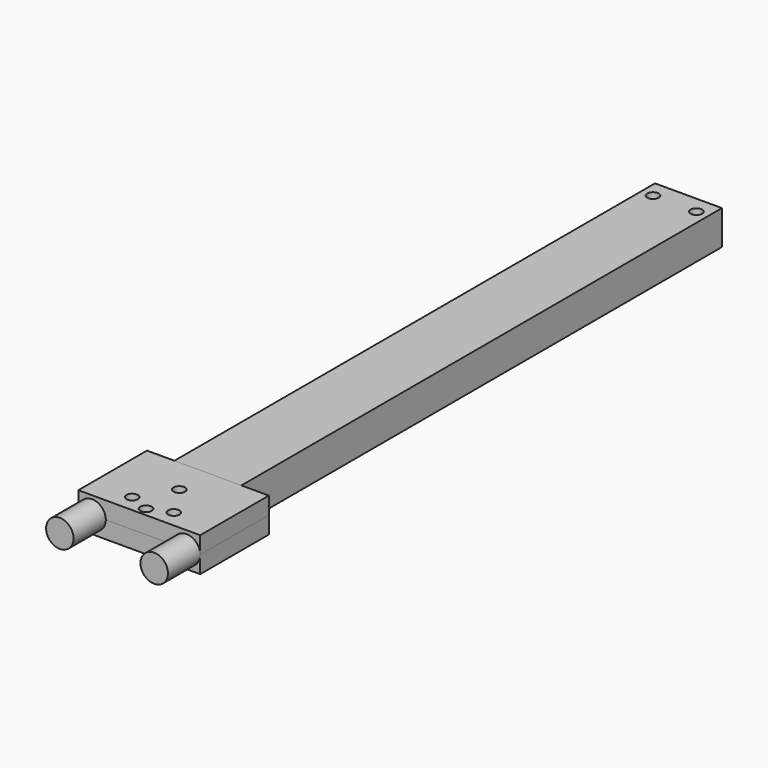
from build123d import *

# Parameters (mm, degrees)
F1_DEPTH   = 11.75
F2_DEPTH   = 25
F3_DEPTH   = 25
F4_DEPTH   = 25
F5_W       = 19.5
F5_H       = 5
F6_DEPTH   = 175
F8_D       = 3.35
F8_DEPTH   = 10
F8_TIP     = 1.0064415369
F8_2_D     = 3.35
F8_2_DEPTH = 10
F8_2_TIP   = 1.0064415369
F8_3_D     = 3.35
F8_3_DEPTH = 10
F8_3_TIP   = 1.0064415369


with BuildPart() as f1:
    # F0 (on Front) → F1 (new body)
    with BuildSketch(Plane.XZ):
        with BuildLine():
            ThreePointArc((-83.867456615, 12.549745962), (-79.867456615, 8.549745962), (-75.867456615, 12.549745962))
            Line((-75.867456615, 12.549745962), (-79.867456615, 12.549745962))
            Line((-79.867456615, 12.549745962), (-83.867456615, 12.549745962))
        make_face()
        with BuildLine():
            Line((-79.867456615, 12.549745962), (-75.867456615, 12.549745962))
            ThreePointArc((-75.867456615, 12.549745962), (-79.867456615, 16.549745962), (-83.867456615, 12.549745962))
            Line((-83.867456615, 12.549745962), (-79.867456615, 12.549745962))
        make_face()
    extrude(amount=F1_DEPTH)


with BuildPart() as f1b:
    # F0 (on Front) → F1, piece 2 (new body)
    with BuildSketch(Plane.XZ):
        with BuildLine():
            ThreePointArc((-103.367456615, 12.549745962), (-107.367456615, 16.549745962), (-111.367456615, 12.549745962))
            Line((-111.367456615, 12.549745962), (-107.367456615, 12.549745962))
            Line((-107.367456615, 12.549745962), (-103.367456615, 12.549745962))
        make_face()
        with BuildLine():
            Line((-107.367456615, 12.549745962), (-111.367456615, 12.549745962))
            ThreePointArc((-111.367456615, 12.549745962), (-107.367456615, 8.549745962), (-103.367456615, 12.549745962))
            Line((-103.367456615, 12.549745962), (-107.367456615, 12.549745962))
        make_face()
    extrude(amount=F1_DEPTH)


with BuildPart() as f2:
    # F0 (on Front) → F2 (new body)
    with BuildSketch(Plane.XZ):
        with BuildLine():
            Line((-75.867456615, 7.549745962), (-75.867456615, 12.549745962))
            ThreePointArc((-75.867456615, 12.549745962), (-79.867456615, 8.549745962), (-83.867456615, 12.549745962))
            Line((-83.867456615, 12.549745962), (-103.367456615, 12.549745962))
            ThreePointArc((-103.367456615, 12.549745962), (-107.367456615, 8.549745962), (-111.367456615, 12.549745962))
            Line((-111.367456615, 12.549745962), (-111.367456615, 7.549745962))
            Line((-111.367456615, 7.549745962), (-75.867456615, 7.549745962))
        make_face()
    extrude(amount=-F2_DEPTH)

    # F8
    with Locations(Plane(origin=(0, 0, 7.549745962), x_dir=(1, 0, 0), z_dir=(0, 0, -1))):
        with Locations((-99.692456615, -5), (-87.542456615, -5), (-99.942456615, -195), (-87.292456615, -195), (-93.617456615, -14.6046723992), (-93.617456615, -2.4546723992)):
            Hole(F8_D / 2, depth=F8_DEPTH)
            with Locations((0, 0, -(F8_DEPTH + F8_TIP / 2))):  # 118° drill point
                Cone(0, F8_D / 2, F8_TIP, mode=Mode.SUBTRACT)


with BuildPart() as f3:
    # F0 (on Front) → F3 (new body)
    with BuildSketch(Plane.XZ):
        with BuildLine():
            Line((-75.867456615, 12.549745962), (-75.867456615, 17.549745962))
            Line((-75.867456615, 17.549745962), (-111.367456615, 17.549745962))
            Line((-111.367456615, 17.549745962), (-111.367456615, 12.549745962))
            ThreePointArc((-111.367456615, 12.549745962), (-107.367456615, 16.549745962), (-103.367456615, 12.549745962))
            Line((-103.367456615, 12.549745962), (-83.867456615, 12.549745962))
            ThreePointArc((-83.867456615, 12.549745962), (-79.867456615, 16.549745962), (-75.867456615, 12.549745962))
        make_face()
    extrude(amount=-F3_DEPTH)

    # F8#2
    with Locations(Plane(origin=(0, 0, 7.549745962), x_dir=(1, 0, 0), z_dir=(0, 0, -1))):
        with Locations((-99.692456615, -5), (-87.542456615, -5), (-99.942456615, -195), (-87.292456615, -195), (-93.617456615, -14.6046723992), (-93.617456615, -2.4546723992)):
            Hole(F8_2_D / 2, depth=F8_2_DEPTH)
            with Locations((0, 0, -(F8_2_DEPTH + F8_2_TIP / 2))):  # 118° drill point
                Cone(0, F8_2_D / 2, F8_2_TIP, mode=Mode.SUBTRACT)


with BuildPart() as f4:
    # F0 (on Front) → F4 (new body)
    with BuildSketch(Plane.XZ):
        with BuildLine():
            ThreePointArc((-83.867456615, 12.549745962), (-79.867456615, 8.549745962), (-75.867456615, 12.549745962))
            Line((-75.867456615, 12.549745962), (-79.867456615, 12.549745962))
            Line((-79.867456615, 12.549745962), (-83.867456615, 12.549745962))
        make_face()
        with BuildLine():
            Line((-79.867456615, 12.549745962), (-75.867456615, 12.549745962))
            ThreePointArc((-75.867456615, 12.549745962), (-79.867456615, 16.549745962), (-83.867456615, 12.549745962))
            Line((-83.867456615, 12.549745962), (-79.867456615, 12.549745962))
        make_face()
    extrude(amount=-F4_DEPTH)


with BuildPart() as f4b:
    # F0 (on Front) → F4, piece 2 (new body)
    with BuildSketch(Plane.XZ):
        with BuildLine():
            ThreePointArc((-103.367456615, 12.549745962), (-107.367456615, 16.549745962), (-111.367456615, 12.549745962))
            Line((-111.367456615, 12.549745962), (-107.367456615, 12.549745962))
            Line((-107.367456615, 12.549745962), (-103.367456615, 12.549745962))
        make_face()
        with BuildLine():
            Line((-107.367456615, 12.549745962), (-111.367456615, 12.549745962))
            ThreePointArc((-111.367456615, 12.549745962), (-107.367456615, 8.549745962), (-103.367456615, 12.549745962))
            Line((-103.367456615, 12.549745962), (-107.367456615, 12.549745962))
        make_face()
    extrude(amount=-F4_DEPTH)


with BuildPart() as f6:
    # F5 (on face) → F6 (new body)
    with BuildSketch(Plane(origin=(0, 25, 0), x_dir=(-1, 0, 0), z_dir=(0, 1, 0))):
        with Locations((93.617456615, 15.049745962)):
            Rectangle(F5_W, F5_H)
        Polygon((100.994568646, 7.549745962), (103.367456615, 7.549745962), (103.367456615, 12.549745962), (83.867456615, 12.549745962), (83.867456615, 7.549745962), align=None)
    extrude(amount=F6_DEPTH)

    # F8#3
    with Locations(Plane(origin=(0, 0, 7.549745962), x_dir=(1, 0, 0), z_dir=(0, 0, -1))):
        with Locations((-99.692456615, -5), (-87.542456615, -5), (-99.942456615, -195), (-87.292456615, -195), (-93.617456615, -14.6046723992), (-93.617456615, -2.4546723992)):
            Hole(F8_3_D / 2, depth=F8_3_DEPTH)
            with Locations((0, 0, -(F8_3_DEPTH + F8_3_TIP / 2))):  # 118° drill point
                Cone(0, F8_3_D / 2, F8_3_TIP, mode=Mode.SUBTRACT)


solid = Compound([f1.part, f1b.part, f2.part, f3.part, f4.part, f4b.part, f6.part])
